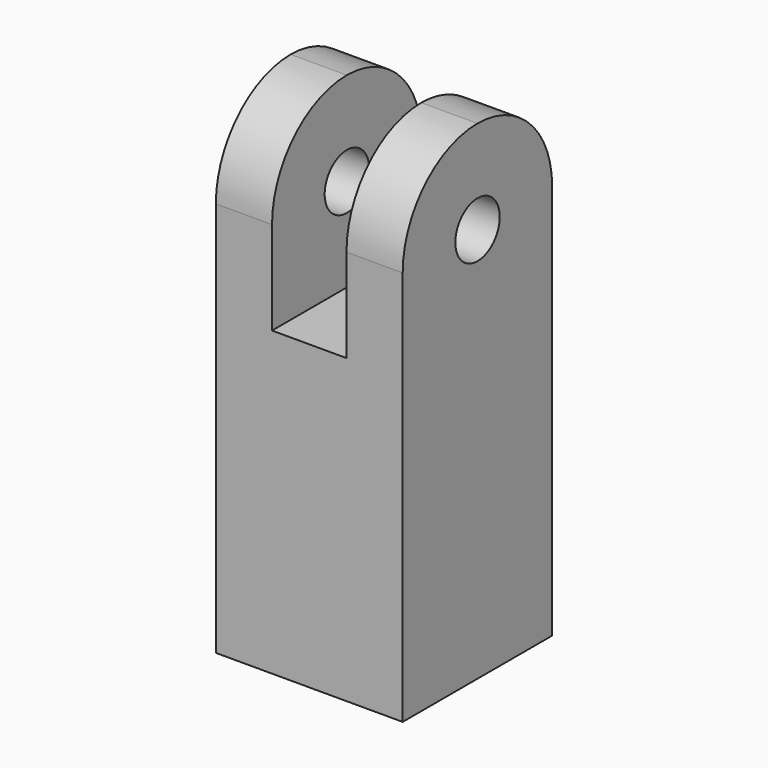
from build123d import *

# Parameters (mm, degrees)
F0_W          = 13.3
F0_H          = 13.3
F0_W_2        = 10.3
F0_H_2        = 10.3
F1_DEPTH      = 20
F2_DEPTH      = 1.5
F3_W          = 4
F3_H          = 13.3
F4_DEPTH      = 13.3
F5_T1_DEPTH   = 37.3
F5_T3_DEPTH   = 37.3
F6_R          = 1.975
F7_DEPTH      = 25
F7_DEPTH_BACK = 25


# Not quite as in the source:
# - a fillet or chamfer that OpenCascade refuses, or shapes differently, is made with other operations: its cross-section is extruded or revolved along the edge and cut away or added


with BuildPart() as f1:
    # F0 (on Top) → F1 (new body)
    with BuildSketch(Plane.XY):
        Rectangle(F0_W, F0_H)
        Rectangle(F0_W_2, F0_H_2, mode=Mode.SUBTRACT)
    extrude(amount=-F1_DEPTH)

    # F0 (on Top) → F2 (join)
    with BuildSketch(Plane.XY):
        Rectangle(F0_W, F0_H)
        Rectangle(F0_W_2, F0_H_2, mode=Mode.SUBTRACT)
        Rectangle(F0_W_2, F0_H_2)
    extrude(amount=F2_DEPTH)

    # F3 (on face) → F4 (join)
    with BuildSketch(Plane.XY.offset(1.5)):
        with Locations((-4.65, 0)):
            Rectangle(F3_W, F3_H)
        with Locations((4.65, 0)):
            Rectangle(F3_W, F3_H)
    extrude(amount=F4_DEPTH)

    # F5: fillet of radius 6.66 on 4 edges, made by hand

    # F5_s2 → F5_t1 (cut)
    with BuildSketch(Plane.YZ.offset(-14)):
        with BuildLine():
            ThreePointArc((-0.01, 14.8), (4.6993311627, 12.8493311627), (6.65, 8.14))
            Line((6.65, 8.14), (6.65, 14.8))
            Line((6.65, 14.8), (-0.01, 14.8))
        make_face()
        with BuildLine():
            ThreePointArc((-6.65, 8.14), (-4.6993311627, 12.8493311627), (0.01, 14.8))
            Line((0.01, 14.8), (-6.65, 14.8))
            Line((-6.65, 14.8), (-6.65, 8.14))
        make_face()
    extrude(amount=F5_T1_DEPTH, mode=Mode.SUBTRACT)

    # F5_s4 → F5_t3 (cut)
    with BuildSketch(Plane.YZ.offset(-23.3)):
        with BuildLine():
            ThreePointArc((-0.01, 14.8), (4.6993311627, 12.8493311627), (6.65, 8.14))
            Line((6.65, 8.14), (6.65, 14.8))
            Line((6.65, 14.8), (-0.01, 14.8))
        make_face()
        with BuildLine():
            ThreePointArc((-6.65, 8.14), (-4.6993311627, 12.8493311627), (0.01, 14.8))
            Line((0.01, 14.8), (-6.65, 14.8))
            Line((-6.65, 14.8), (-6.65, 8.14))
        make_face()
    extrude(amount=F5_T3_DEPTH, mode=Mode.SUBTRACT)

    # F6 (on face) → F7 (cut, two sides)
    with BuildSketch(Plane.YZ.offset(6.65)) as f7_sk:
        with Locations((0.01, 8.14)):
            Circle(F6_R)
    extrude(amount=-F7_DEPTH, mode=Mode.SUBTRACT)
    extrude(f7_sk.sketch, amount=F7_DEPTH_BACK, mode=Mode.SUBTRACT)


solid = f1.part
